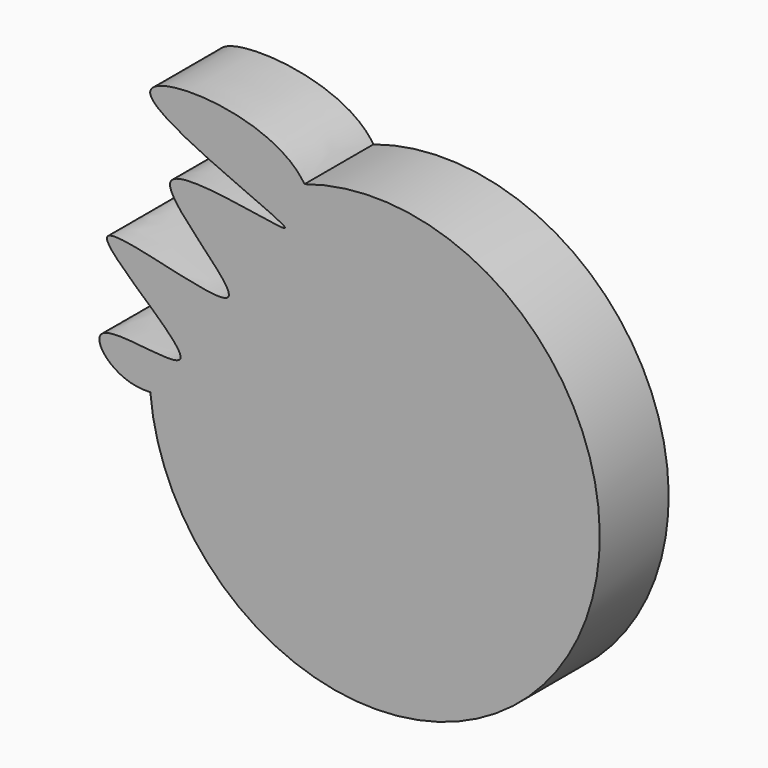
from build123d import *

# Parameters (mm, degrees)
F1_DEPTH = 25


with BuildPart() as f1:
    # F0 (on Front) → F1 (new body)
    with BuildSketch(Plane.XZ):
        with BuildLine():
            add(Edge.make_bspline(
                [(-30.0269797444, 67.7023455501), (-17.3247250732, 47.7716972688), (-52.8505344727, 1.6762077404), (-74.7841745615, 0)],
                knots=[0.8336548496, 0.8336548496, 0.8336548496, 0.8336548496, 1, 1, 1, 1], degree=3))
            ThreePointArc((-74.7841745615, 0), (44.8387298443, -30.435852405), (-30.0269797444, 67.7023455501))
        make_face()
        with BuildLine():
            add(Edge.make_bspline(
                [(-74.7841745615, 0), (-84.938008863, -0.7759740555), (-100.449294077, 17.9539630279), (-45.1391808821, 1.8432996539), (-114.3971690671, 49.8216503582), (-26.5098819208, 17.7417174135), (-94.1339625418, 67.9277197493), (-1.7673344801, 44.6479731779), (-112.3457165496, 83.1229447559), (-39.5437321689, 82.6347374964), (-30.0269797444, 67.7023455501)],
                knots=[0, 0, 0, 0, 0.0770068756, 0.1649618246, 0.2695951364, 0.3793769086, 0.4793425991, 0.5856745846, 0.7090261396, 0.8336548496, 0.8336548496, 0.8336548496, 0.8336548496], degree=3))
            add(Edge.make_bspline(
                [(-30.0269797444, 67.7023455501), (-17.3247250732, 47.7716972688), (-52.8505344727, 1.6762077404), (-74.7841745615, 0)],
                knots=[0.8336548496, 0.8336548496, 0.8336548496, 0.8336548496, 1, 1, 1, 1], degree=3))
        make_face()
    extrude(amount=F1_DEPTH)


solid = f1.part
